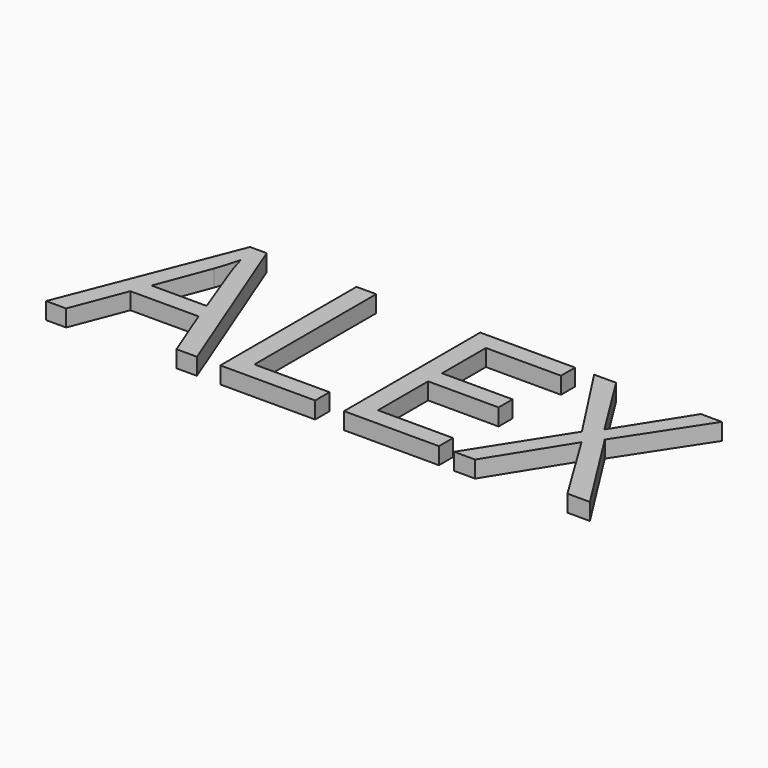
from build123d import *

# Parameters (mm, degrees)
F0_TEXT_SIZE = 36.0178321393
F1_DEPTH     = 2.54


# Not quite as in the source:
# - Text() gives the source's letters only with a copy of the font that has no kerning and outlines rounded to 1/6400 em; it was checked with that copy


with BuildPart() as f1:
    # F0 (on Top) → F1 (new body)
    with BuildSketch(Plane.XY):
        with Locations((-23.6455779523, 0)):
            Text('ALEX', F0_TEXT_SIZE, font='Open Sans', text_align=(TextAlign.LEFT, TextAlign.BOTTOM))
    extrude(amount=F1_DEPTH)


solid = f1.part
